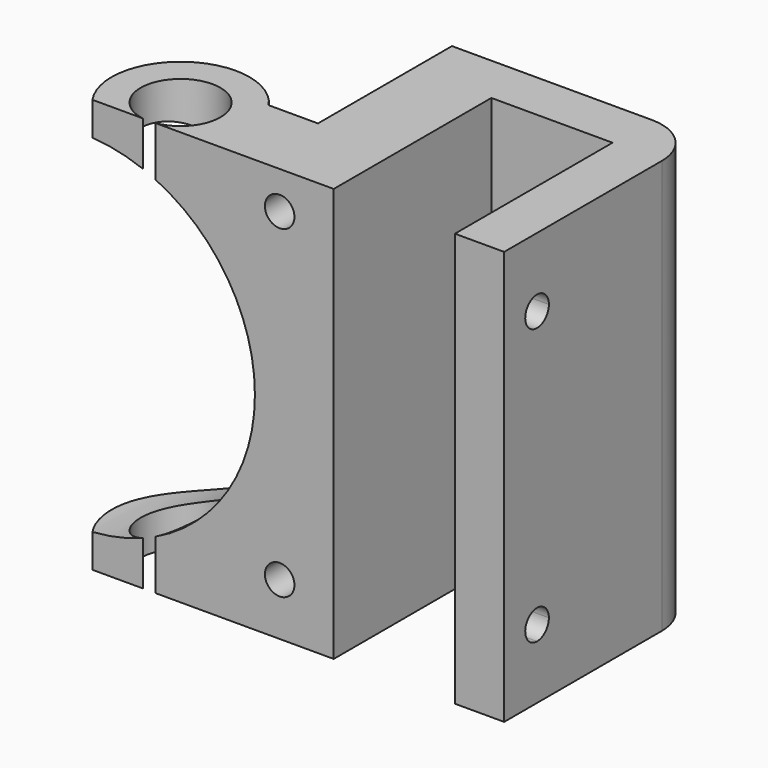
from build123d import *

# Parameters (mm, degrees)
F1_DEPTH      = 42
F2_R          = 1.5
F3_DEPTH      = 25.001
F3_DEPTH_BACK = 90
F6_DEPTH      = 25


# Not quite as in the source:
# - an extrude ends at something that could not be found from the text; its depth is read off the source's solid


with BuildPart() as f1:
    # F0 (on Top) → F1 (new body)
    with BuildSketch(Plane.XY):
        with BuildLine():
            Line((-12.622932768, 0), (-7.5127989985, 0))
            Line((-7.5127989985, 0), (-7.5127989985, 8))
            ThreePointArc((-7.5127989985, 8), (-17.257361645, 9.7445626465), (-19.0019242916, 0))
            Line((-19.0019242916, 0), (-13.8917905221, 0))
            ThreePointArc((-13.8917905221, 0), (-15.8872915916, 7.0799299466), (-9.207361645, 4))
            ThreePointArc((-9.207361645, 4), (-10.1774316984, 1.3700700534), (-12.622932768, 0))
        make_face()
        with BuildLine():
            ThreePointArc((-6.257361645, 4), (-6.5785916039, 1.9038056538), (-7.5127989985, 0))
            Line((-7.5127989985, 0), (-2.5127989985, 0))
            Line((-2.5127989985, 0), (-2.5127989985, 8))
            Line((-2.5127989985, 8), (-7.5127989985, 8))
            ThreePointArc((-7.5127989985, 8), (-6.5785916039, 6.0961943462), (-6.257361645, 4))
        make_face()
        with BuildLine():
            Line((-7.5127989985, 8), (-7.5127989985, 0))
            ThreePointArc((-7.5127989985, 0), (-6.5785916039, 1.9038056538), (-6.257361645, 4))
            ThreePointArc((-6.257361645, 4), (-6.5785916039, 6.0961943462), (-7.5127989985, 8))
        make_face()
        with BuildLine():
            Line((-2.5127989985, 8), (-2.5127989985, 0))
            Line((-2.5127989985, 0), (5.4872010015, 0))
            Line((5.4872010015, 0), (5.4872010015, 20))
            Line((5.4872010015, 20), (17.7872010015, 20))
            Line((17.7872010015, 20), (17.7872010015, 0))
            Line((17.7872010015, 0), (22.7872010015, 0))
            Line((22.7872010015, 0), (22.7872010015, 20))
            ThreePointArc((22.7872010015, 20), (21.3227349074, 23.5355339059), (17.7872010015, 25))
            Line((17.7872010015, 25), (-2.5127989985, 25))
            Line((-2.5127989985, 25), (-2.5127989985, 8))
        make_face()
    extrude(amount=F1_DEPTH)

    # F2 (on Front) → F3 (cut, two sides)
    with BuildSketch(Plane.XZ) as f3_sk:
        with BuildLine():
            Line((-20.1659295708, 21), (-20.1659295708, 38.6531305723))
            ThreePointArc((-20.1659295708, 38.6531305723), (-37.8190601431, 21), (-20.1659295708, 3.3468694277))
            Line((-20.1659295708, 3.3468694277), (-20.1659295708, 21))
        make_face()
        with BuildLine():
            ThreePointArc((-20.1659295708, 3.3468694277), (-7.683281234, 8.5173516632), (-2.5127989985, 21))
            Line((-2.5127989985, 21), (-20.1659295708, 21))
            Line((-20.1659295708, 21), (-20.1659295708, 3.3468694277))
        make_face()
        with Locations((0, 38.2)):
            Circle(F2_R)
        with Locations((0, 5.3)):
            Circle(F2_R)
        with BuildLine():
            Line((-20.1659295708, 21), (-2.5127989985, 21))
            ThreePointArc((-2.5127989985, 21), (-7.683281234, 33.4826483368), (-20.1659295708, 38.6531305723))
            Line((-20.1659295708, 38.6531305723), (-20.1659295708, 21))
        make_face()
    extrude(amount=-F3_DEPTH, mode=Mode.SUBTRACT)
    extrude(f3_sk.sketch, amount=F3_DEPTH_BACK, mode=Mode.SUBTRACT)

    # F5 (on offset) → F6 (cut)
    with BuildSketch(Plane.YZ.offset(10)):
        with BuildLine():
            ThreePointArc((4.1718953289, 5.5), (5.2325555007, 5.9393398282), (5.6718953289, 7))
            ThreePointArc((5.6718953289, 7), (3.1112351571, 8.0606601718), (4.1718953289, 5.5))
        make_face()
        with BuildLine():
            ThreePointArc((4.1718953289, 36.5), (3.1112351571, 33.9393398282), (5.6718953289, 35))
            ThreePointArc((5.6718953289, 35), (5.2325555007, 36.0606601718), (4.1718953289, 36.5))
        make_face()
    extrude(amount=F6_DEPTH, mode=Mode.SUBTRACT)


solid = f1.part
